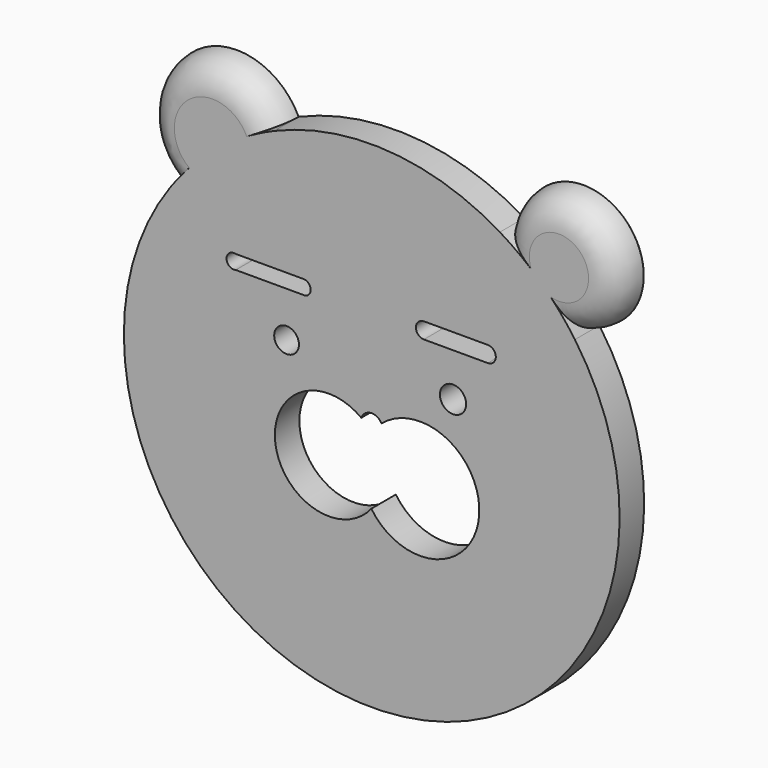
from build123d import *

# Parameters (mm, degrees)
F0_R        = 2.017634
F0_R_2      = 2.136586
F1_DEPTH    = 5
F2_T4_ANGLE = 359.64
F2_S5_R     = 40.434853
F2_T6_DEPTH = 16
F3_T4_ANGLE = 334.187533
F3_S5_R     = 40.434853
F3_T6_DEPTH = 19


# Not quite as in the source:
# - a fillet or chamfer that OpenCascade refuses, or shapes differently, is made with other operations: its cross-section is extruded or revolved along the edge and cut away or added


with BuildPart() as f1:
    # F0 (on Front) → F1 (new body)
    with BuildSketch(Plane.XZ):
        with BuildLine():
            ThreePointArc((-15.926206, 37.166293), (-33.028098, 41.004742), (-32.920731, 23.47771))
            ThreePointArc((-32.920731, 23.47771), (-0.190207, -40.434406), (33.140151, 23.166954))
            ThreePointArc((33.140151, 23.166954), (37.249636, 39.829607), (20.899072, 34.615114))
            ThreePointArc((20.899072, 34.615114), (2.794544, 40.338169), (-15.926206, 37.166293))
        make_face()
        with BuildLine():
            ThreePointArc((-0.07357, -11.922027), (-15.7306, -7.603253), (-1.708722, 0.593169))
            ThreePointArc((-1.708722, 0.593169), (-0.144497, 1.80297), (1.592441, 0.857737))
            ThreePointArc((1.592441, 0.857737), (17.461414, -7.709469), (-0.07357, -11.922027))
        make_face(mode=Mode.SUBTRACT)
        with Locations((-13.894406, 7.804544)):
            Circle(F0_R, mode=Mode.SUBTRACT)
        with Locations((13.257022, 8.11134)):
            Circle(F0_R_2, mode=Mode.SUBTRACT)
        with BuildLine():
            ThreePointArc((-22.177892, 15.167643), (-23.686122, 16.318127), (-22.177892, 17.468611))
            Line((-22.177892, 17.468611), (-11.133244, 17.468611))
            ThreePointArc((-11.133244, 17.468611), (-9.972579, 16.45243), (-10.826448, 15.167643))
            Line((-10.826448, 15.167643), (-22.177892, 15.167643))
        make_face(mode=Mode.SUBTRACT)
        with BuildLine():
            ThreePointArc((8.501687, 15.167643), (7.197805, 16.471525), (8.501687, 17.775407))
            Line((8.501687, 17.775407), (18.932743, 17.775407))
            ThreePointArc((18.932743, 17.775407), (20.236625, 16.471525), (18.932743, 15.167643))
            Line((18.932743, 15.167643), (8.501687, 15.167643))
        make_face(mode=Mode.SUBTRACT)
    extrude(amount=F1_DEPTH)

    # F2: fillet of radius 5 on 1 edges, made by hand


with BuildPart() as f2_tool2:
    # F2_s3 → F2_t4 (revolve)
    with BuildSketch(Plane(origin=(0.102867, 0, -0.0956), x_dir=(0, 1, 0), z_dir=(-0.732508, 0, 0.680758))):
        with BuildLine():
            ThreePointArc((0, -34.867737), (-3.535534, -36.332203), (-5, -39.867737))
            Line((-5, -39.867737), (-5, -34.867737))
            Line((-5, -34.867737), (0, -34.867737))
        make_face()
    revolve(axis=Axis((30.533206, -5, 32.647985), (0, -1, 0)), revolution_arc=F2_T4_ANGLE)

    # F2_s5 → F2_t6 (cut, symmetric)
    with BuildSketch(Plane.XZ.offset(2.5)):
        Circle(F2_S5_R)
    extrude(amount=F2_T6_DEPTH, both=True, mode=Mode.SUBTRACT)


with BuildPart() as f1_1:
    add(f1.part)

    # F2_t1: cut F2_tool2
    add(f2_tool2.part, mode=Mode.SUBTRACT)

    # F3: fillet of radius 5 on 1 edges, made by hand


with BuildPart() as f3_tool2:
    # F3_s3 → F3_t4 (revolve)
    with BuildSketch(Plane(origin=(5.731373, 0, 7.271945), x_dir=(0, 1, 0), z_dir=(-0.619003, 0, -0.785389))):
        with BuildLine():
            ThreePointArc((0, -29.208934), (-3.535534, -30.6734), (-5, -34.208934))
            Line((-5, -34.208934), (-5, -29.208934))
            Line((-5, -29.208934), (0, -29.208934))
        make_face()
    revolve(axis=Axis((-26.003741, -5, 32.283927), (0, -1, 0)), revolution_arc=F3_T4_ANGLE)

    # F3_s5 → F3_t6 (cut, symmetric)
    with BuildSketch(Plane.XZ.offset(2.5)):
        Circle(F3_S5_R)
    extrude(amount=F3_T6_DEPTH, both=True, mode=Mode.SUBTRACT)


with BuildPart() as f1_2:
    add(f1_1.part)

    # F3_t1: cut F3_tool2
    add(f3_tool2.part, mode=Mode.SUBTRACT)


solid = f1_2.part
